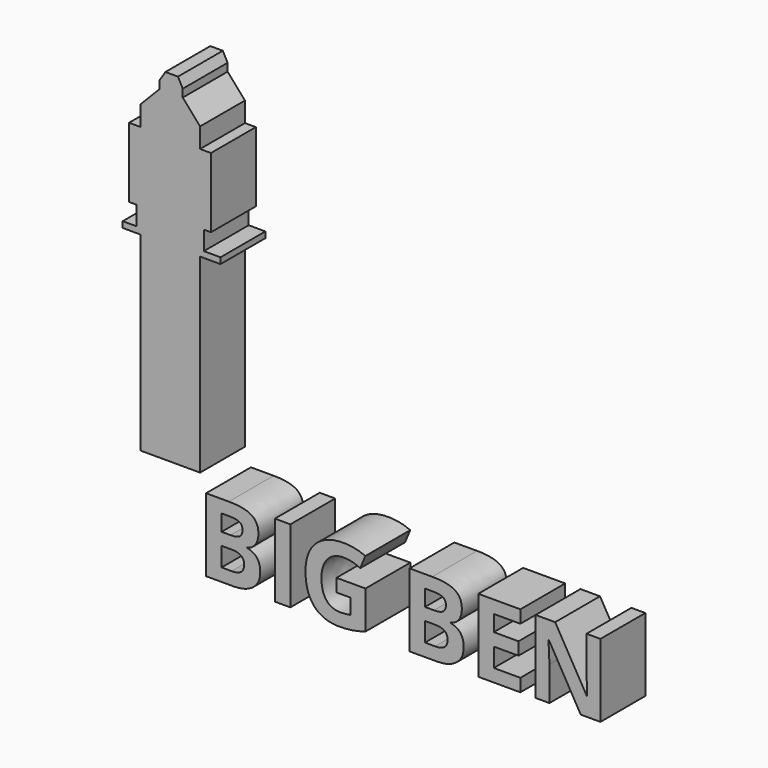
from build123d import *

# Parameters (mm, degrees)
F0_TEXT_SIZE = 45.6453197532
F1_DEPTH     = 25


# Not quite as in the source:
# - Text() gives the source's letters only with a copy of the font that has no kerning and outlines rounded to 1/6400 em; it was checked with that copy


with BuildPart() as f1:
    # F0 (on Front) → F1 (new body)
    with BuildSketch(Plane.XZ):
        Polygon((28.3189024776, -67.42528826), (28.3189024776, -152.2258222103), (54.9144782126, -152.2258222103), (54.9144782126, -67.42528826), (64.0123337507, -67.42528826), (64.0123337507, -64.7478848696), (56.5824210644, -64.7478848696), (56.5824210644, -56.2948323786), (59.7666688263, -56.2948323786), (59.7666688263, -25.1939687878), (54.9144782126, -25.1939687878), (54.9144782126, -16.3256749511), (47.1813045442, -7.531081792), (47.1813045442, -4.043571651), (45.0584702194, 0), (39.4481271505, 0), (36.8704013526, -4.043571651), (36.8704013526, -7.531081792), (28.3189024776, -16.3256749511), (28.3189024776, -25.1939687878), (23.2393629849, -25.1939687878), (23.2393629849, -56.2948323786), (26.5886876732, -56.2948323786), (26.5886876732, -64.7478848696), (20.4139985144, -64.7478848696), (20.4139985144, -67.42528826), align=None)
        with Locations((53.4746982157, -192.0239329338)):
            Text('BIG BEN', F0_TEXT_SIZE, font='Open Sans', font_style=FontStyle.BOLD, text_align=(TextAlign.LEFT, TextAlign.BOTTOM))
    extrude(amount=F1_DEPTH)


solid = f1.part
